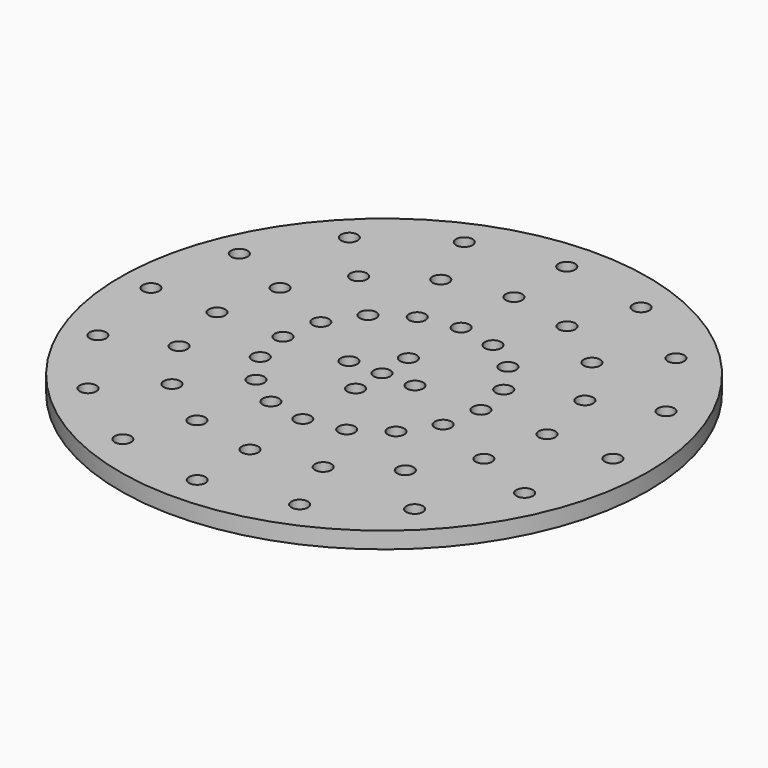
from build123d import *

# Parameters (mm, degrees)
F0_R     = 101.6
F0_R_2   = 3.175
F1_DEPTH = 6.35


# Not quite as in the source:
# - the program builds the solid bodies; features that only make, move or delete a surface that nothing else refers to are left out


with BuildPart() as f1:
    # F0 (on Top) → F1 (new body)
    with BuildSketch(Plane.XY):
        with Locations((1.0160004022, -0.2540000132)):
            Circle(F0_R)
        with Locations((-62.8617928475, -62.8617928475)):
            Circle(F0_R_2, mode=Mode.SUBTRACT)
        with Locations((-34.0205571373, -82.1328904403)):
            Circle(F0_R_2, mode=Mode.SUBTRACT)
        with Locations((0, -88.9)):
            Circle(F0_R_2, mode=Mode.SUBTRACT)
        with Locations((-24.3003979552, -58.6663503145)):
            Circle(F0_R_2, mode=Mode.SUBTRACT)
        with Locations((0, -63.5)):
            Circle(F0_R_2, mode=Mode.SUBTRACT)
        with Locations((-82.1328904403, -34.0205571373)):
            Circle(F0_R_2, mode=Mode.SUBTRACT)
        with Locations((-58.6663503145, -24.3003979552)):
            Circle(F0_R_2, mode=Mode.SUBTRACT)
        with Locations((-44.9012806053, -44.9012806053)):
            Circle(F0_R_2, mode=Mode.SUBTRACT)
        with Locations((-26.9407683632, -26.9407683632)):
            Circle(F0_R_2, mode=Mode.SUBTRACT)
        with Locations((-14.5802387731, -35.1998101887)):
            Circle(F0_R_2, mode=Mode.SUBTRACT)
        with Locations((0, -38.1)):
            Circle(F0_R_2, mode=Mode.SUBTRACT)
        with Locations((-35.1998101887, -14.5802387731)):
            Circle(F0_R_2, mode=Mode.SUBTRACT)
        with Locations((0, -12.7)):
            Circle(F0_R_2, mode=Mode.SUBTRACT)
        with Locations((34.0205571373, -82.1328904403)):
            Circle(F0_R_2, mode=Mode.SUBTRACT)
        with Locations((24.3003979552, -58.6663503145)):
            Circle(F0_R_2, mode=Mode.SUBTRACT)
        with Locations((62.8617928475, -62.8617928475)):
            Circle(F0_R_2, mode=Mode.SUBTRACT)
        with Locations((14.5802387731, -35.1998101887)):
            Circle(F0_R_2, mode=Mode.SUBTRACT)
        with Locations((44.9012806053, -44.9012806053)):
            Circle(F0_R_2, mode=Mode.SUBTRACT)
        with Locations((26.9407683632, -26.9407683632)):
            Circle(F0_R_2, mode=Mode.SUBTRACT)
        with Locations((35.1998101887, -14.5802387731)):
            Circle(F0_R_2, mode=Mode.SUBTRACT)
        with Locations((82.1328904403, -34.0205571373)):
            Circle(F0_R_2, mode=Mode.SUBTRACT)
        with Locations((58.6663503145, -24.3003979552)):
            Circle(F0_R_2, mode=Mode.SUBTRACT)
        with Locations((-88.9, 0)):
            Circle(F0_R_2, mode=Mode.SUBTRACT)
        with Locations((-63.5, 0)):
            Circle(F0_R_2, mode=Mode.SUBTRACT)
        with Locations((-58.6663503145, 24.3003979552)):
            Circle(F0_R_2, mode=Mode.SUBTRACT)
        with Locations((-82.1328904403, 34.0205571373)):
            Circle(F0_R_2, mode=Mode.SUBTRACT)
        with Locations((-38.1, 0)):
            Circle(F0_R_2, mode=Mode.SUBTRACT)
        with Locations((-35.1998101887, 14.5802387731)):
            Circle(F0_R_2, mode=Mode.SUBTRACT)
        with Locations((-12.7, 0)):
            Circle(F0_R_2, mode=Mode.SUBTRACT)
        Circle(F0_R_2, mode=Mode.SUBTRACT)
        with Locations((0, 12.7)):
            Circle(F0_R_2, mode=Mode.SUBTRACT)
        with Locations((-26.9407683632, 26.9407683632)):
            Circle(F0_R_2, mode=Mode.SUBTRACT)
        with Locations((-44.9012806053, 44.9012806053)):
            Circle(F0_R_2, mode=Mode.SUBTRACT)
        with Locations((-14.5802387731, 35.1998101887)):
            Circle(F0_R_2, mode=Mode.SUBTRACT)
        with Locations((0, 38.1)):
            Circle(F0_R_2, mode=Mode.SUBTRACT)
        with Locations((-62.8617928475, 62.8617928475)):
            Circle(F0_R_2, mode=Mode.SUBTRACT)
        with Locations((-24.3003979552, 58.6663503145)):
            Circle(F0_R_2, mode=Mode.SUBTRACT)
        with Locations((0, 63.5)):
            Circle(F0_R_2, mode=Mode.SUBTRACT)
        with Locations((-34.0205571373, 82.1328904403)):
            Circle(F0_R_2, mode=Mode.SUBTRACT)
        with Locations((0, 88.9)):
            Circle(F0_R_2, mode=Mode.SUBTRACT)
        with Locations((12.7, 0)):
            Circle(F0_R_2, mode=Mode.SUBTRACT)
        with Locations((38.1, 0)):
            Circle(F0_R_2, mode=Mode.SUBTRACT)
        with Locations((35.1998101887, 14.5802387731)):
            Circle(F0_R_2, mode=Mode.SUBTRACT)
        with Locations((14.5802387731, 35.1998101887)):
            Circle(F0_R_2, mode=Mode.SUBTRACT)
        with Locations((26.9407683632, 26.9407683632)):
            Circle(F0_R_2, mode=Mode.SUBTRACT)
        with Locations((44.9012806053, 44.9012806053)):
            Circle(F0_R_2, mode=Mode.SUBTRACT)
        with Locations((63.5, 0)):
            Circle(F0_R_2, mode=Mode.SUBTRACT)
        with Locations((58.6663503145, 24.3003979552)):
            Circle(F0_R_2, mode=Mode.SUBTRACT)
        with Locations((88.9, 0)):
            Circle(F0_R_2, mode=Mode.SUBTRACT)
        with Locations((82.1328904403, 34.0205571373)):
            Circle(F0_R_2, mode=Mode.SUBTRACT)
        with Locations((24.3003979552, 58.6663503145)):
            Circle(F0_R_2, mode=Mode.SUBTRACT)
        with Locations((34.0205571373, 82.1328904403)):
            Circle(F0_R_2, mode=Mode.SUBTRACT)
        with Locations((62.8617928475, 62.8617928475)):
            Circle(F0_R_2, mode=Mode.SUBTRACT)
    extrude(amount=F1_DEPTH)


solid = f1.part
